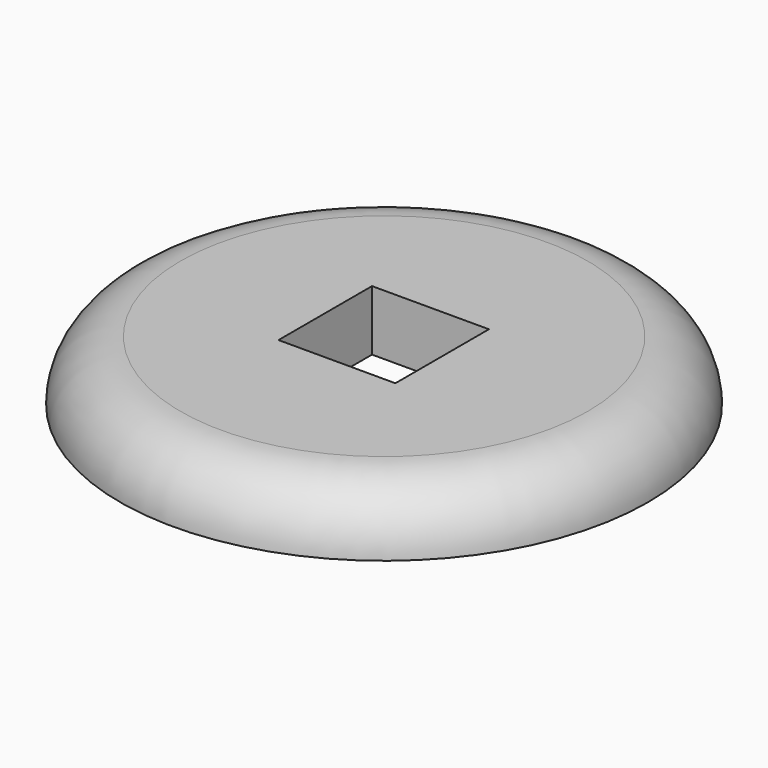
from build123d import *

# Parameters (mm, degrees)
F0_R     = 35
F0_W     = 15.5
F0_H     = 15.5
F1_DEPTH = 8
F2_R     = 7.99999


# Not quite as in the source:
# - a fillet or chamfer is up to 0.001 mm smaller than in the source, because OpenCascade refuses the exact size


with BuildPart() as f1:
    # F0 (on Top) → F1 (new body)
    with BuildSketch(Plane.XY):
        Circle(F0_R)
        with Locations((-0.25, 0.25)):
            Rectangle(F0_W, F0_H, mode=Mode.SUBTRACT)
    extrude(amount=F1_DEPTH)

    # F2 (radius 8 in the source; OpenCascade refuses exactly that, so slightly less here)
    f2_edges = [f1.edges().sort_by_distance(p)[0] for p in [
        (-35, 0, 8),
    ]]
    fillet(f2_edges, radius=F2_R)


solid = f1.part
